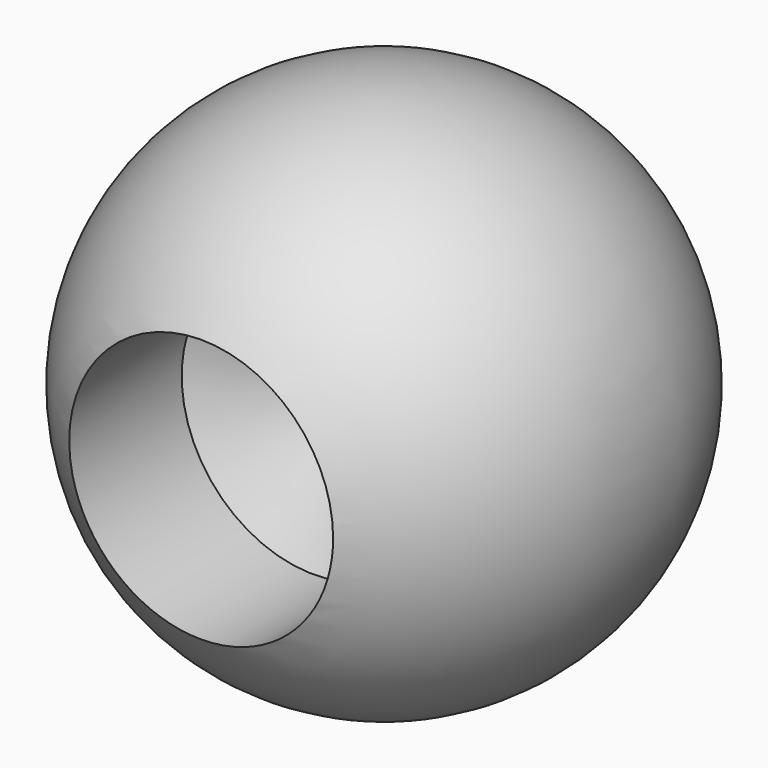
from build123d import *

# Parameters (mm, degrees)
F4_D     = 9.525
F4_DEPTH = 6.35
F4_TIP   = 2.8615986981


# Not quite as in the source:
# - a length typed as a fraction of an inch, garbled in the dataset ("3 / 203.2 mm" for 3/8 in), is restored


with BuildPart() as f1:
    # F0 (on Front) → F1 (revolve)
    with BuildSketch(Plane.XZ):
        with BuildLine():
            Line((0, 9.525), (0, -9.525))
            ThreePointArc((0, -9.525), (9.525, 0), (0, 9.525))
        make_face()
    revolve(axis=Axis((0, 0, 0), (0, 0, -1)))

    # F4 (one way)
    with BuildSketch(Plane.XZ.offset(9.525)):
        with Locations((0, 0)):
            Circle(F4_D / 2)
    extrude(amount=-F4_DEPTH, mode=Mode.SUBTRACT)
    with Locations(Plane.XZ.offset(9.525)):
        with Locations((0, 0)):
            with Locations((0, 0, -(F4_DEPTH + F4_TIP / 2))):  # 118° drill point
                Cone(0, F4_D / 2, F4_TIP, mode=Mode.SUBTRACT)


solid = f1.part
